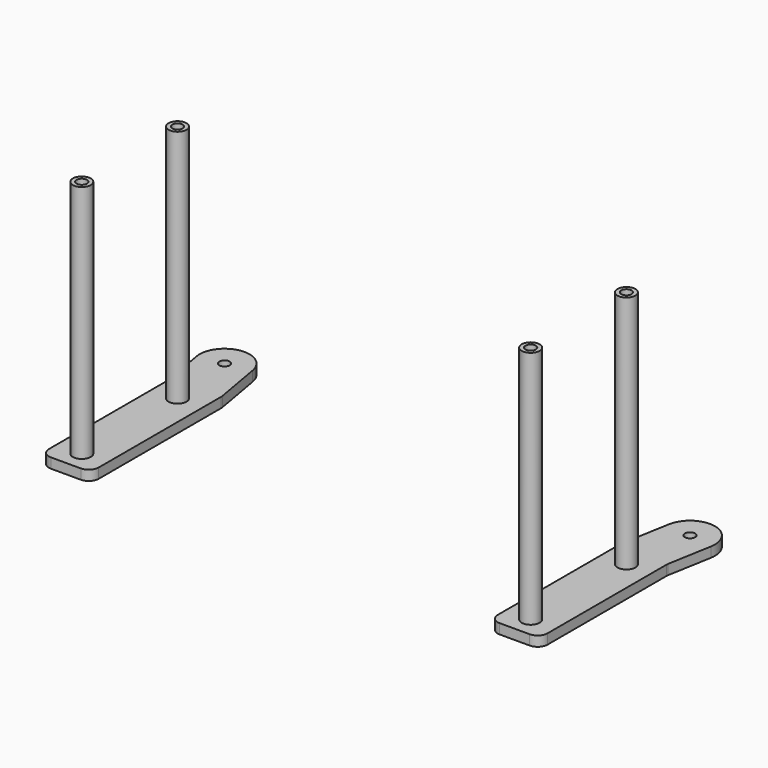
from build123d import *

# Parameters (mm, degrees)
F0_R     = 3.302
F1_DEPTH = 6.35
F2_R     = 5.715
F2_R_2   = 3.302
F3_DEPTH = 152.4


# Not quite as in the source:
# - a feature names something its author has since deleted; it is built from what else it names


with BuildPart() as f1:
    # F0 (on Top) → F1 (new body)
    with BuildSketch(Plane.XY):
        with BuildLine():
            ThreePointArc((-132.5168345954, 34.0652888097), (-150.9073224949, 46.9424470683), (-163.7844807535, 28.5519591688))
            Line((-163.7844807535, 28.5519591688), (-158.8464707684, 0.5471129148))
            ThreePointArc((-158.8464707684, 0.5471129148), (-158.7741636671, -0.0021140469), (-158.75, -0.5555530134))
            Line((-158.75, -0.5555530134), (-158.75, -95.25))
            ThreePointArc((-158.75, -95.25), (-156.8901280605, -99.7401280605), (-152.4, -101.6))
            Line((-152.4, -101.6), (-133.35, -101.6))
            ThreePointArc((-133.35, -101.6), (-128.8598719395, -99.7401280605), (-127, -95.25))
            Line((-127, -95.25), (-127, 0))
            Line((-127, 0), (-127, 2.2222120536))
            ThreePointArc((-127, 2.2222120536), (-127.0241636671, 2.77565102), (-127.0964707684, 3.3248779817))
            Line((-127.0964707684, 3.3248779817), (-132.5168345954, 34.0652888097))
        make_face()
        with Locations((-142.875, -88.9)):
            Circle(F0_R, mode=Mode.SUBTRACT)
        with Locations((-142.875, -12.7)):
            Circle(F0_R, mode=Mode.SUBTRACT)
        with Locations((-148.1506576745, 31.3086239893)):
            Circle(F0_R, mode=Mode.SUBTRACT)
    extrude(amount=F1_DEPTH)


with BuildPart() as f1b:
    # F0 (on Top) → F1, piece 2 (new body)
    with BuildSketch(Plane.XY):
        with BuildLine():
            ThreePointArc((163.7844807535, 28.5519591688), (150.9073224949, 46.9424470683), (132.5168345954, 34.0652888097))
            Line((132.5168345954, 34.0652888097), (127.0964707684, 3.3248779817))
            ThreePointArc((127.0964707684, 3.3248779817), (127.0241636671, 2.77565102), (127, 2.2222120536))
            Line((127, 2.2222120536), (127, 0))
            Line((127, 0), (127, -95.25))
            ThreePointArc((127, -95.25), (128.8598719395, -99.7401280605), (133.35, -101.6))
            Line((133.35, -101.6), (152.4, -101.6))
            ThreePointArc((152.4, -101.6), (156.8901280605, -99.7401280605), (158.75, -95.25))
            Line((158.75, -95.25), (158.75, -0.5555530134))
            ThreePointArc((158.75, -0.5555530134), (158.7741636671, -0.0021140469), (158.8464707684, 0.5471129148))
            Line((158.8464707684, 0.5471129148), (163.7844807535, 28.5519591688))
        make_face()
        with Locations((142.875, -88.9)):
            Circle(F0_R, mode=Mode.SUBTRACT)
        with Locations((142.875, -12.7)):
            Circle(F0_R, mode=Mode.SUBTRACT)
        with Locations((148.1506576745, 31.3086239893)):
            Circle(F0_R, mode=Mode.SUBTRACT)
    extrude(amount=F1_DEPTH)


with BuildPart() as f3:
    # F2 (on face) → F3 (new body)
    with BuildSketch(Plane.XY.offset(6.35)):
        with Locations((-142.875, -12.7)):
            Circle(F2_R)
        with Locations((-142.875, -12.7)):
            Circle(F2_R_2, mode=Mode.SUBTRACT)
    extrude(amount=F3_DEPTH)


with BuildPart() as f3b:
    # F2 (on face) → F3, piece 2 (new body)
    with BuildSketch(Plane.XY.offset(6.35)):
        with Locations((-142.875, -88.9)):
            Circle(F2_R)
        with Locations((-142.875, -88.9)):
            Circle(F2_R_2, mode=Mode.SUBTRACT)
    extrude(amount=F3_DEPTH)


with BuildPart() as f3c:
    # F2 (on face) → F3, piece 3 (new body)
    with BuildSketch(Plane.XY.offset(6.35)):
        with Locations((142.875, -12.7)):
            Circle(F2_R)
        with Locations((142.875, -12.7)):
            Circle(F2_R_2, mode=Mode.SUBTRACT)
    extrude(amount=F3_DEPTH)


with BuildPart() as f3d:
    # F2 (on face) → F3, piece 4 (new body)
    with BuildSketch(Plane.XY.offset(6.35)):
        with Locations((142.875, -88.9)):
            Circle(F2_R)
        with Locations((142.875, -88.9)):
            Circle(F2_R_2, mode=Mode.SUBTRACT)
    extrude(amount=F3_DEPTH)


solid = Compound([f1.part, f1b.part, f3.part, f3b.part, f3c.part, f3d.part])
